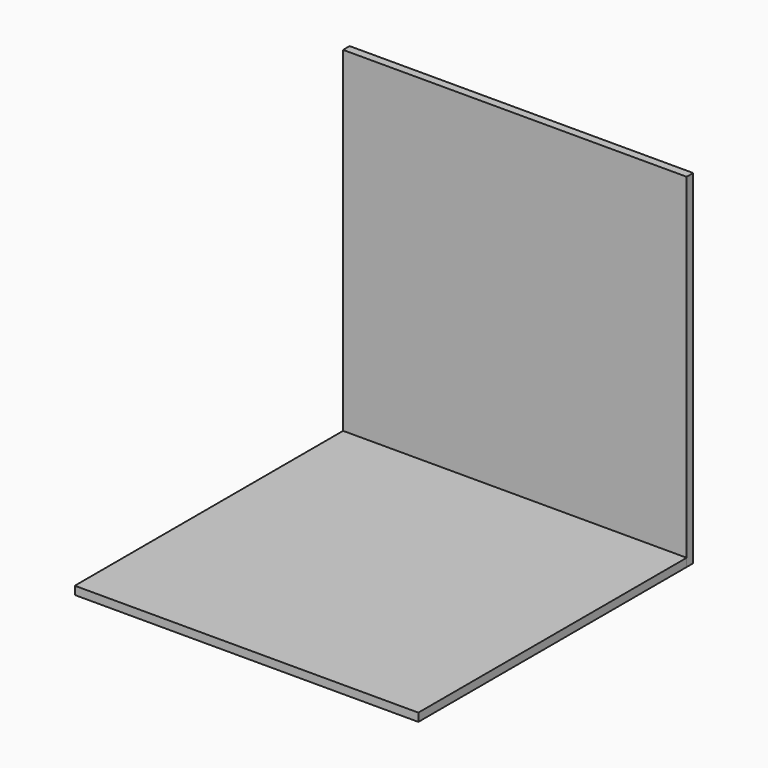
from build123d import *

# Parameters (mm, degrees)
F0_W     = 133.35
F0_H     = 133.35
F1_DEPTH = 3.175
F2_W     = 133.35
F2_H     = 3.175
F3_DEPTH = 133.35
F4_W     = 25.4
F4_H     = 3.175
F5_DEPTH = 3.175


with BuildPart() as f1:
    # F0 (on Front) → F1 (new body)
    with BuildSketch(Plane.XZ):
        Rectangle(F0_W, F0_H)
    extrude(amount=F1_DEPTH)


with BuildPart() as f3:
    # F2 (on face) → F3 (new body)
    with BuildSketch(Plane.XZ):
        with Locations((0, -65.0875)):
            Rectangle(F2_W, F2_H)
    extrude(amount=F3_DEPTH)

    # F4 (on face) → F5 (cut)
    with BuildSketch(Plane(origin=(0, 0, -66.675), x_dir=(1, 0, 0), z_dir=(0, 0, -1))):
        with Locations((-53.975, 1.5875)):
            Rectangle(F4_W, F4_H)
        with Locations((-7.62, 1.5875)):
            Rectangle(F4_W, F4_H)
        with Locations((38.735, 1.5875)):
            Rectangle(F4_W, F4_H)
    extrude(amount=-F5_DEPTH, mode=Mode.SUBTRACT)

    # F6: cut F1
    add(f1.part, mode=Mode.SUBTRACT)


solid = Compound([f1.part, f3.part])
